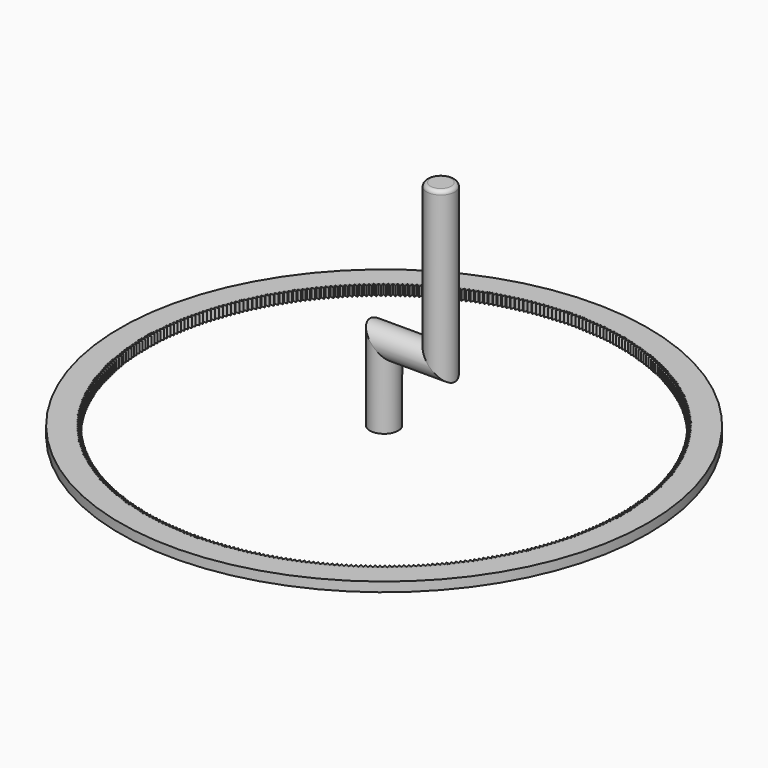
from build123d import *

# Parameters (mm, degrees)
F1_R     = 7.5
F3_R     = 2
F4_R     = 139.7
F6_DEPTH = 5
F7_COUNT = 399


# Not quite as in the source:
# - a feature names something its author has since deleted; it is built from what else it names


with BuildPart() as f2:
    # F2: sweep along a path in F0
    with BuildLine(Plane.XZ) as f2_path:
        Line((0, 0), (0, 40))
        Line((0, 40), (30, 40))
        Line((30, 40), (30, 123))
    # F1 (on Top) → F2 (sweep)
    with BuildSketch(Plane.XY):
        Circle(F1_R)
    sweep(path=f2_path.line, transition=Transition.RIGHT)

    # F3
    f3_edges = [f2.edges().sort_by_distance(p)[0] for p in [
        (22.5, 0, 123),
    ]]
    fillet(f3_edges, radius=F3_R)


with BuildPart() as f6:
    # F4 (on Top) → F6 (new body)
    with BuildSketch(Plane.XY):
        Circle(F4_R)
        with BuildLine():
            Line((127, 4.9999837018), (127, 0))
            Line((127, 0), (127, -4.9999837018))
            Line((127, -4.9999837018), (126.9015372759, -4.9999837018))
            ThreePointArc((126.9015372759, -4.9999837018), (89.8025612107, -89.8025612107), (4.9999837018, -126.9015372759))
            Line((4.9999837018, -126.9015372759), (4.9999837018, -127))
            Line((4.9999837018, -127), (0, -127))
            Line((0, -127), (-4.9999837018, -127))
            Line((-4.9999837018, -127), (-4.9999837018, -126.9015372759))
            ThreePointArc((-4.9999837018, -126.9015372759), (-89.8025612107, -89.8025612107), (-126.9015372759, -4.9999837018))
            Line((-126.9015372759, -4.9999837018), (-127, -4.9999837018))
            Line((-127, -4.9999837018), (-127, 0))
            Line((-127, 0), (-127, 4.9999837018))
            Line((-127, 4.9999837018), (-126.9015372759, 4.9999837018))
            ThreePointArc((-126.9015372759, 4.9999837018), (-89.8025612107, 89.8025612107), (-4.9999837018, 126.9015372759))
            Line((-4.9999837018, 126.9015372759), (-4.9999837018, 127))
            Line((-4.9999837018, 127), (0, 127))
            Line((0, 127), (4.9999837018, 127))
            Line((4.9999837018, 127), (4.9999837018, 126.9015372759))
            ThreePointArc((4.9999837018, 126.9015372759), (89.8025612107, 89.8025612107), (126.9015372759, 4.9999837018))
            Line((126.9015372759, 4.9999837018), (127, 4.9999837018))
        make_face(mode=Mode.SUBTRACT)
        with BuildLine():
            Line((4.9999837018, -127), (4.9999837018, -126.9015372759))
            ThreePointArc((4.9999837018, -126.9015372759), (2.5004765509, -126.9753819329), (0, -127))
            Line((0, -127), (4.9999837018, -127))
        make_face()
        with BuildLine():
            Line((-4.9999837018, -127), (0, -127))
            ThreePointArc((0, -127), (-2.5004765509, -126.9753819329), (-4.9999837018, -126.9015372759))
            Line((-4.9999837018, -126.9015372759), (-4.9999837018, -127))
        make_face()
    extrude(amount=-F6_DEPTH)


with BuildPart() as f6b:
    # F4 (on Top) → F6, piece 2 (new body)
    with BuildSketch(Plane.XY):
        Polygon((-4.75e-08, -125.2242034363), (-1.0000000475, -126.9562542439), (0.9999999525, -126.9562542439), align=None)
    extrude(amount=-F6_DEPTH)


with BuildPart() as f7_1:
    # F7: instance of F6b
    add(f6b.part.rotate(Axis((0, 0, 36.9798913598), (0, 0, 1)), 1 * 360 / F7_COUNT))


with BuildPart() as f7_2:
    # F7: instance of F6b
    add(f6b.part.rotate(Axis((0, 0, 36.9798913598), (0, 0, 1)), 2 * 360 / F7_COUNT))


with BuildPart() as f7_3:
    # F7: instance of F6b
    add(f6b.part.rotate(Axis((0, 0, 36.9798913598), (0, 0, 1)), 3 * 360 / F7_COUNT))


with BuildPart() as f7_4:
    # F7: instance of F6b
    add(f6b.part.rotate(Axis((0, 0, 36.9798913598), (0, 0, 1)), 4 * 360 / F7_COUNT))


with BuildPart() as f7_5:
    # F7: instance of F6b
    add(f6b.part.rotate(Axis((0, 0, 36.9798913598), (0, 0, 1)), 5 * 360 / F7_COUNT))


with BuildPart() as f7_6:
    # F7: instance of F6b
    add(f6b.part.rotate(Axis((0, 0, 36.9798913598), (0, 0, 1)), 6 * 360 / F7_COUNT))


with BuildPart() as f7_7:
    # F7: instance of F6b
    add(f6b.part.rotate(Axis((0, 0, 36.9798913598), (0, 0, 1)), 7 * 360 / F7_COUNT))


with BuildPart() as f7_8:
    # F7: instance of F6b
    add(f6b.part.rotate(Axis((0, 0, 36.9798913598), (0, 0, 1)), 8 * 360 / F7_COUNT))


with BuildPart() as f7_9:
    # F7: instance of F6b
    add(f6b.part.rotate(Axis((0, 0, 36.9798913598), (0, 0, 1)), 9 * 360 / F7_COUNT))


with BuildPart() as f7_10:
    # F7: instance of F6b
    add(f6b.part.rotate(Axis((0, 0, 36.9798913598), (0, 0, 1)), 10 * 360 / F7_COUNT))


with BuildPart() as f7_11:
    # F7: instance of F6b
    add(f6b.part.rotate(Axis((0, 0, 36.9798913598), (0, 0, 1)), 11 * 360 / F7_COUNT))


with BuildPart() as f7_12:
    # F7: instance of F6b
    add(f6b.part.rotate(Axis((0, 0, 36.9798913598), (0, 0, 1)), 12 * 360 / F7_COUNT))


with BuildPart() as f7_13:
    # F7: instance of F6b
    add(f6b.part.rotate(Axis((0, 0, 36.9798913598), (0, 0, 1)), 13 * 360 / F7_COUNT))


with BuildPart() as f7_14:
    # F7: instance of F6b
    add(f6b.part.rotate(Axis((0, 0, 36.9798913598), (0, 0, 1)), 14 * 360 / F7_COUNT))


with BuildPart() as f7_15:
    # F7: instance of F6b
    add(f6b.part.rotate(Axis((0, 0, 36.9798913598), (0, 0, 1)), 15 * 360 / F7_COUNT))


with BuildPart() as f7_16:
    # F7: instance of F6b
    add(f6b.part.rotate(Axis((0, 0, 36.9798913598), (0, 0, 1)), 16 * 360 / F7_COUNT))


with BuildPart() as f7_17:
    # F7: instance of F6b
    add(f6b.part.rotate(Axis((0, 0, 36.9798913598), (0, 0, 1)), 17 * 360 / F7_COUNT))


with BuildPart() as f7_18:
    # F7: instance of F6b
    add(f6b.part.rotate(Axis((0, 0, 36.9798913598), (0, 0, 1)), 18 * 360 / F7_COUNT))


with BuildPart() as f7_19:
    # F7: instance of F6b
    add(f6b.part.rotate(Axis((0, 0, 36.9798913598), (0, 0, 1)), 19 * 360 / F7_COUNT))


with BuildPart() as f7_20:
    # F7: instance of F6b
    add(f6b.part.rotate(Axis((0, 0, 36.9798913598), (0, 0, 1)), 20 * 360 / F7_COUNT))


with BuildPart() as f7_21:
    # F7: instance of F6b
    add(f6b.part.rotate(Axis((0, 0, 36.9798913598), (0, 0, 1)), 21 * 360 / F7_COUNT))


with BuildPart() as f7_22:
    # F7: instance of F6b
    add(f6b.part.rotate(Axis((0, 0, 36.9798913598), (0, 0, 1)), 22 * 360 / F7_COUNT))


with BuildPart() as f7_23:
    # F7: instance of F6b
    add(f6b.part.rotate(Axis((0, 0, 36.9798913598), (0, 0, 1)), 23 * 360 / F7_COUNT))


with BuildPart() as f7_24:
    # F7: instance of F6b
    add(f6b.part.rotate(Axis((0, 0, 36.9798913598), (0, 0, 1)), 24 * 360 / F7_COUNT))


with BuildPart() as f7_25:
    # F7: instance of F6b
    add(f6b.part.rotate(Axis((0, 0, 36.9798913598), (0, 0, 1)), 25 * 360 / F7_COUNT))


with BuildPart() as f7_26:
    # F7: instance of F6b
    add(f6b.part.rotate(Axis((0, 0, 36.9798913598), (0, 0, 1)), 26 * 360 / F7_COUNT))


with BuildPart() as f7_27:
    # F7: instance of F6b
    add(f6b.part.rotate(Axis((0, 0, 36.9798913598), (0, 0, 1)), 27 * 360 / F7_COUNT))


with BuildPart() as f7_28:
    # F7: instance of F6b
    add(f6b.part.rotate(Axis((0, 0, 36.9798913598), (0, 0, 1)), 28 * 360 / F7_COUNT))


with BuildPart() as f7_29:
    # F7: instance of F6b
    add(f6b.part.rotate(Axis((0, 0, 36.9798913598), (0, 0, 1)), 29 * 360 / F7_COUNT))


with BuildPart() as f7_30:
    # F7: instance of F6b
    add(f6b.part.rotate(Axis((0, 0, 36.9798913598), (0, 0, 1)), 30 * 360 / F7_COUNT))


with BuildPart() as f7_31:
    # F7: instance of F6b
    add(f6b.part.rotate(Axis((0, 0, 36.9798913598), (0, 0, 1)), 31 * 360 / F7_COUNT))


with BuildPart() as f7_32:
    # F7: instance of F6b
    add(f6b.part.rotate(Axis((0, 0, 36.9798913598), (0, 0, 1)), 32 * 360 / F7_COUNT))


with BuildPart() as f7_33:
    # F7: instance of F6b
    add(f6b.part.rotate(Axis((0, 0, 36.9798913598), (0, 0, 1)), 33 * 360 / F7_COUNT))


with BuildPart() as f7_34:
    # F7: instance of F6b
    add(f6b.part.rotate(Axis((0, 0, 36.9798913598), (0, 0, 1)), 34 * 360 / F7_COUNT))


with BuildPart() as f7_35:
    # F7: instance of F6b
    add(f6b.part.rotate(Axis((0, 0, 36.9798913598), (0, 0, 1)), 35 * 360 / F7_COUNT))


with BuildPart() as f7_36:
    # F7: instance of F6b
    add(f6b.part.rotate(Axis((0, 0, 36.9798913598), (0, 0, 1)), 36 * 360 / F7_COUNT))


with BuildPart() as f7_37:
    # F7: instance of F6b
    add(f6b.part.rotate(Axis((0, 0, 36.9798913598), (0, 0, 1)), 37 * 360 / F7_COUNT))


with BuildPart() as f7_38:
    # F7: instance of F6b
    add(f6b.part.rotate(Axis((0, 0, 36.9798913598), (0, 0, 1)), 38 * 360 / F7_COUNT))


with BuildPart() as f7_39:
    # F7: instance of F6b
    add(f6b.part.rotate(Axis((0, 0, 36.9798913598), (0, 0, 1)), 39 * 360 / F7_COUNT))


with BuildPart() as f7_40:
    # F7: instance of F6b
    add(f6b.part.rotate(Axis((0, 0, 36.9798913598), (0, 0, 1)), 40 * 360 / F7_COUNT))


with BuildPart() as f7_41:
    # F7: instance of F6b
    add(f6b.part.rotate(Axis((0, 0, 36.9798913598), (0, 0, 1)), 41 * 360 / F7_COUNT))


with BuildPart() as f7_42:
    # F7: instance of F6b
    add(f6b.part.rotate(Axis((0, 0, 36.9798913598), (0, 0, 1)), 42 * 360 / F7_COUNT))


with BuildPart() as f7_43:
    # F7: instance of F6b
    add(f6b.part.rotate(Axis((0, 0, 36.9798913598), (0, 0, 1)), 43 * 360 / F7_COUNT))


with BuildPart() as f7_44:
    # F7: instance of F6b
    add(f6b.part.rotate(Axis((0, 0, 36.9798913598), (0, 0, 1)), 44 * 360 / F7_COUNT))


with BuildPart() as f7_45:
    # F7: instance of F6b
    add(f6b.part.rotate(Axis((0, 0, 36.9798913598), (0, 0, 1)), 45 * 360 / F7_COUNT))


with BuildPart() as f7_46:
    # F7: instance of F6b
    add(f6b.part.rotate(Axis((0, 0, 36.9798913598), (0, 0, 1)), 46 * 360 / F7_COUNT))


with BuildPart() as f7_47:
    # F7: instance of F6b
    add(f6b.part.rotate(Axis((0, 0, 36.9798913598), (0, 0, 1)), 47 * 360 / F7_COUNT))


with BuildPart() as f7_48:
    # F7: instance of F6b
    add(f6b.part.rotate(Axis((0, 0, 36.9798913598), (0, 0, 1)), 48 * 360 / F7_COUNT))


with BuildPart() as f7_49:
    # F7: instance of F6b
    add(f6b.part.rotate(Axis((0, 0, 36.9798913598), (0, 0, 1)), 49 * 360 / F7_COUNT))


with BuildPart() as f7_50:
    # F7: instance of F6b
    add(f6b.part.rotate(Axis((0, 0, 36.9798913598), (0, 0, 1)), 50 * 360 / F7_COUNT))


with BuildPart() as f7_51:
    # F7: instance of F6b
    add(f6b.part.rotate(Axis((0, 0, 36.9798913598), (0, 0, 1)), 51 * 360 / F7_COUNT))


with BuildPart() as f7_52:
    # F7: instance of F6b
    add(f6b.part.rotate(Axis((0, 0, 36.9798913598), (0, 0, 1)), 52 * 360 / F7_COUNT))


with BuildPart() as f7_53:
    # F7: instance of F6b
    add(f6b.part.rotate(Axis((0, 0, 36.9798913598), (0, 0, 1)), 53 * 360 / F7_COUNT))


with BuildPart() as f7_54:
    # F7: instance of F6b
    add(f6b.part.rotate(Axis((0, 0, 36.9798913598), (0, 0, 1)), 54 * 360 / F7_COUNT))


with BuildPart() as f7_55:
    # F7: instance of F6b
    add(f6b.part.rotate(Axis((0, 0, 36.9798913598), (0, 0, 1)), 55 * 360 / F7_COUNT))


with BuildPart() as f7_56:
    # F7: instance of F6b
    add(f6b.part.rotate(Axis((0, 0, 36.9798913598), (0, 0, 1)), 56 * 360 / F7_COUNT))


with BuildPart() as f7_57:
    # F7: instance of F6b
    add(f6b.part.rotate(Axis((0, 0, 36.9798913598), (0, 0, 1)), 57 * 360 / F7_COUNT))


with BuildPart() as f7_58:
    # F7: instance of F6b
    add(f6b.part.rotate(Axis((0, 0, 36.9798913598), (0, 0, 1)), 58 * 360 / F7_COUNT))


with BuildPart() as f7_59:
    # F7: instance of F6b
    add(f6b.part.rotate(Axis((0, 0, 36.9798913598), (0, 0, 1)), 59 * 360 / F7_COUNT))


with BuildPart() as f7_60:
    # F7: instance of F6b
    add(f6b.part.rotate(Axis((0, 0, 36.9798913598), (0, 0, 1)), 60 * 360 / F7_COUNT))


with BuildPart() as f7_61:
    # F7: instance of F6b
    add(f6b.part.rotate(Axis((0, 0, 36.9798913598), (0, 0, 1)), 61 * 360 / F7_COUNT))


with BuildPart() as f7_62:
    # F7: instance of F6b
    add(f6b.part.rotate(Axis((0, 0, 36.9798913598), (0, 0, 1)), 62 * 360 / F7_COUNT))


with BuildPart() as f7_63:
    # F7: instance of F6b
    add(f6b.part.rotate(Axis((0, 0, 36.9798913598), (0, 0, 1)), 63 * 360 / F7_COUNT))


with BuildPart() as f7_64:
    # F7: instance of F6b
    add(f6b.part.rotate(Axis((0, 0, 36.9798913598), (0, 0, 1)), 64 * 360 / F7_COUNT))


with BuildPart() as f7_65:
    # F7: instance of F6b
    add(f6b.part.rotate(Axis((0, 0, 36.9798913598), (0, 0, 1)), 65 * 360 / F7_COUNT))


with BuildPart() as f7_66:
    # F7: instance of F6b
    add(f6b.part.rotate(Axis((0, 0, 36.9798913598), (0, 0, 1)), 66 * 360 / F7_COUNT))


with BuildPart() as f7_67:
    # F7: instance of F6b
    add(f6b.part.rotate(Axis((0, 0, 36.9798913598), (0, 0, 1)), 67 * 360 / F7_COUNT))


with BuildPart() as f7_68:
    # F7: instance of F6b
    add(f6b.part.rotate(Axis((0, 0, 36.9798913598), (0, 0, 1)), 68 * 360 / F7_COUNT))


with BuildPart() as f7_69:
    # F7: instance of F6b
    add(f6b.part.rotate(Axis((0, 0, 36.9798913598), (0, 0, 1)), 69 * 360 / F7_COUNT))


with BuildPart() as f7_70:
    # F7: instance of F6b
    add(f6b.part.rotate(Axis((0, 0, 36.9798913598), (0, 0, 1)), 70 * 360 / F7_COUNT))


with BuildPart() as f7_71:
    # F7: instance of F6b
    add(f6b.part.rotate(Axis((0, 0, 36.9798913598), (0, 0, 1)), 71 * 360 / F7_COUNT))


with BuildPart() as f7_72:
    # F7: instance of F6b
    add(f6b.part.rotate(Axis((0, 0, 36.9798913598), (0, 0, 1)), 72 * 360 / F7_COUNT))


with BuildPart() as f7_73:
    # F7: instance of F6b
    add(f6b.part.rotate(Axis((0, 0, 36.9798913598), (0, 0, 1)), 73 * 360 / F7_COUNT))


with BuildPart() as f7_74:
    # F7: instance of F6b
    add(f6b.part.rotate(Axis((0, 0, 36.9798913598), (0, 0, 1)), 74 * 360 / F7_COUNT))


with BuildPart() as f7_75:
    # F7: instance of F6b
    add(f6b.part.rotate(Axis((0, 0, 36.9798913598), (0, 0, 1)), 75 * 360 / F7_COUNT))


with BuildPart() as f7_76:
    # F7: instance of F6b
    add(f6b.part.rotate(Axis((0, 0, 36.9798913598), (0, 0, 1)), 76 * 360 / F7_COUNT))


with BuildPart() as f7_77:
    # F7: instance of F6b
    add(f6b.part.rotate(Axis((0, 0, 36.9798913598), (0, 0, 1)), 77 * 360 / F7_COUNT))


with BuildPart() as f7_78:
    # F7: instance of F6b
    add(f6b.part.rotate(Axis((0, 0, 36.9798913598), (0, 0, 1)), 78 * 360 / F7_COUNT))


with BuildPart() as f7_79:
    # F7: instance of F6b
    add(f6b.part.rotate(Axis((0, 0, 36.9798913598), (0, 0, 1)), 79 * 360 / F7_COUNT))


with BuildPart() as f7_80:
    # F7: instance of F6b
    add(f6b.part.rotate(Axis((0, 0, 36.9798913598), (0, 0, 1)), 80 * 360 / F7_COUNT))


with BuildPart() as f7_81:
    # F7: instance of F6b
    add(f6b.part.rotate(Axis((0, 0, 36.9798913598), (0, 0, 1)), 81 * 360 / F7_COUNT))


with BuildPart() as f7_82:
    # F7: instance of F6b
    add(f6b.part.rotate(Axis((0, 0, 36.9798913598), (0, 0, 1)), 82 * 360 / F7_COUNT))


with BuildPart() as f7_83:
    # F7: instance of F6b
    add(f6b.part.rotate(Axis((0, 0, 36.9798913598), (0, 0, 1)), 83 * 360 / F7_COUNT))


with BuildPart() as f7_84:
    # F7: instance of F6b
    add(f6b.part.rotate(Axis((0, 0, 36.9798913598), (0, 0, 1)), 84 * 360 / F7_COUNT))


with BuildPart() as f7_85:
    # F7: instance of F6b
    add(f6b.part.rotate(Axis((0, 0, 36.9798913598), (0, 0, 1)), 85 * 360 / F7_COUNT))


with BuildPart() as f7_86:
    # F7: instance of F6b
    add(f6b.part.rotate(Axis((0, 0, 36.9798913598), (0, 0, 1)), 86 * 360 / F7_COUNT))


with BuildPart() as f7_87:
    # F7: instance of F6b
    add(f6b.part.rotate(Axis((0, 0, 36.9798913598), (0, 0, 1)), 87 * 360 / F7_COUNT))


with BuildPart() as f7_88:
    # F7: instance of F6b
    add(f6b.part.rotate(Axis((0, 0, 36.9798913598), (0, 0, 1)), 88 * 360 / F7_COUNT))


with BuildPart() as f7_89:
    # F7: instance of F6b
    add(f6b.part.rotate(Axis((0, 0, 36.9798913598), (0, 0, 1)), 89 * 360 / F7_COUNT))


with BuildPart() as f7_90:
    # F7: instance of F6b
    add(f6b.part.rotate(Axis((0, 0, 36.9798913598), (0, 0, 1)), 90 * 360 / F7_COUNT))


with BuildPart() as f7_91:
    # F7: instance of F6b
    add(f6b.part.rotate(Axis((0, 0, 36.9798913598), (0, 0, 1)), 91 * 360 / F7_COUNT))


with BuildPart() as f7_92:
    # F7: instance of F6b
    add(f6b.part.rotate(Axis((0, 0, 36.9798913598), (0, 0, 1)), 92 * 360 / F7_COUNT))


with BuildPart() as f7_93:
    # F7: instance of F6b
    add(f6b.part.rotate(Axis((0, 0, 36.9798913598), (0, 0, 1)), 93 * 360 / F7_COUNT))


with BuildPart() as f7_94:
    # F7: instance of F6b
    add(f6b.part.rotate(Axis((0, 0, 36.9798913598), (0, 0, 1)), 94 * 360 / F7_COUNT))


with BuildPart() as f7_95:
    # F7: instance of F6b
    add(f6b.part.rotate(Axis((0, 0, 36.9798913598), (0, 0, 1)), 95 * 360 / F7_COUNT))


with BuildPart() as f7_96:
    # F7: instance of F6b
    add(f6b.part.rotate(Axis((0, 0, 36.9798913598), (0, 0, 1)), 96 * 360 / F7_COUNT))


with BuildPart() as f7_97:
    # F7: instance of F6b
    add(f6b.part.rotate(Axis((0, 0, 36.9798913598), (0, 0, 1)), 97 * 360 / F7_COUNT))


with BuildPart() as f7_98:
    # F7: instance of F6b
    add(f6b.part.rotate(Axis((0, 0, 36.9798913598), (0, 0, 1)), 98 * 360 / F7_COUNT))


with BuildPart() as f7_99:
    # F7: instance of F6b
    add(f6b.part.rotate(Axis((0, 0, 36.9798913598), (0, 0, 1)), 99 * 360 / F7_COUNT))


with BuildPart() as f7_100:
    # F7: instance of F6b
    add(f6b.part.rotate(Axis((0, 0, 36.9798913598), (0, 0, 1)), 100 * 360 / F7_COUNT))


with BuildPart() as f7_101:
    # F7: instance of F6b
    add(f6b.part.rotate(Axis((0, 0, 36.9798913598), (0, 0, 1)), 101 * 360 / F7_COUNT))


with BuildPart() as f7_102:
    # F7: instance of F6b
    add(f6b.part.rotate(Axis((0, 0, 36.9798913598), (0, 0, 1)), 102 * 360 / F7_COUNT))


with BuildPart() as f7_103:
    # F7: instance of F6b
    add(f6b.part.rotate(Axis((0, 0, 36.9798913598), (0, 0, 1)), 103 * 360 / F7_COUNT))


with BuildPart() as f7_104:
    # F7: instance of F6b
    add(f6b.part.rotate(Axis((0, 0, 36.9798913598), (0, 0, 1)), 104 * 360 / F7_COUNT))


with BuildPart() as f7_105:
    # F7: instance of F6b
    add(f6b.part.rotate(Axis((0, 0, 36.9798913598), (0, 0, 1)), 105 * 360 / F7_COUNT))


with BuildPart() as f7_106:
    # F7: instance of F6b
    add(f6b.part.rotate(Axis((0, 0, 36.9798913598), (0, 0, 1)), 106 * 360 / F7_COUNT))


with BuildPart() as f7_107:
    # F7: instance of F6b
    add(f6b.part.rotate(Axis((0, 0, 36.9798913598), (0, 0, 1)), 107 * 360 / F7_COUNT))


with BuildPart() as f7_108:
    # F7: instance of F6b
    add(f6b.part.rotate(Axis((0, 0, 36.9798913598), (0, 0, 1)), 108 * 360 / F7_COUNT))


with BuildPart() as f7_109:
    # F7: instance of F6b
    add(f6b.part.rotate(Axis((0, 0, 36.9798913598), (0, 0, 1)), 109 * 360 / F7_COUNT))


with BuildPart() as f7_110:
    # F7: instance of F6b
    add(f6b.part.rotate(Axis((0, 0, 36.9798913598), (0, 0, 1)), 110 * 360 / F7_COUNT))


with BuildPart() as f7_111:
    # F7: instance of F6b
    add(f6b.part.rotate(Axis((0, 0, 36.9798913598), (0, 0, 1)), 111 * 360 / F7_COUNT))


with BuildPart() as f7_112:
    # F7: instance of F6b
    add(f6b.part.rotate(Axis((0, 0, 36.9798913598), (0, 0, 1)), 112 * 360 / F7_COUNT))


with BuildPart() as f7_113:
    # F7: instance of F6b
    add(f6b.part.rotate(Axis((0, 0, 36.9798913598), (0, 0, 1)), 113 * 360 / F7_COUNT))


with BuildPart() as f7_114:
    # F7: instance of F6b
    add(f6b.part.rotate(Axis((0, 0, 36.9798913598), (0, 0, 1)), 114 * 360 / F7_COUNT))


with BuildPart() as f7_115:
    # F7: instance of F6b
    add(f6b.part.rotate(Axis((0, 0, 36.9798913598), (0, 0, 1)), 115 * 360 / F7_COUNT))


with BuildPart() as f7_116:
    # F7: instance of F6b
    add(f6b.part.rotate(Axis((0, 0, 36.9798913598), (0, 0, 1)), 116 * 360 / F7_COUNT))


with BuildPart() as f7_117:
    # F7: instance of F6b
    add(f6b.part.rotate(Axis((0, 0, 36.9798913598), (0, 0, 1)), 117 * 360 / F7_COUNT))


with BuildPart() as f7_118:
    # F7: instance of F6b
    add(f6b.part.rotate(Axis((0, 0, 36.9798913598), (0, 0, 1)), 118 * 360 / F7_COUNT))


with BuildPart() as f7_119:
    # F7: instance of F6b
    add(f6b.part.rotate(Axis((0, 0, 36.9798913598), (0, 0, 1)), 119 * 360 / F7_COUNT))


with BuildPart() as f7_120:
    # F7: instance of F6b
    add(f6b.part.rotate(Axis((0, 0, 36.9798913598), (0, 0, 1)), 120 * 360 / F7_COUNT))


with BuildPart() as f7_121:
    # F7: instance of F6b
    add(f6b.part.rotate(Axis((0, 0, 36.9798913598), (0, 0, 1)), 121 * 360 / F7_COUNT))


with BuildPart() as f7_122:
    # F7: instance of F6b
    add(f6b.part.rotate(Axis((0, 0, 36.9798913598), (0, 0, 1)), 122 * 360 / F7_COUNT))


with BuildPart() as f7_123:
    # F7: instance of F6b
    add(f6b.part.rotate(Axis((0, 0, 36.9798913598), (0, 0, 1)), 123 * 360 / F7_COUNT))


with BuildPart() as f7_124:
    # F7: instance of F6b
    add(f6b.part.rotate(Axis((0, 0, 36.9798913598), (0, 0, 1)), 124 * 360 / F7_COUNT))


with BuildPart() as f7_125:
    # F7: instance of F6b
    add(f6b.part.rotate(Axis((0, 0, 36.9798913598), (0, 0, 1)), 125 * 360 / F7_COUNT))


with BuildPart() as f7_126:
    # F7: instance of F6b
    add(f6b.part.rotate(Axis((0, 0, 36.9798913598), (0, 0, 1)), 126 * 360 / F7_COUNT))


with BuildPart() as f7_127:
    # F7: instance of F6b
    add(f6b.part.rotate(Axis((0, 0, 36.9798913598), (0, 0, 1)), 127 * 360 / F7_COUNT))


with BuildPart() as f7_128:
    # F7: instance of F6b
    add(f6b.part.rotate(Axis((0, 0, 36.9798913598), (0, 0, 1)), 128 * 360 / F7_COUNT))


with BuildPart() as f7_129:
    # F7: instance of F6b
    add(f6b.part.rotate(Axis((0, 0, 36.9798913598), (0, 0, 1)), 129 * 360 / F7_COUNT))


with BuildPart() as f7_130:
    # F7: instance of F6b
    add(f6b.part.rotate(Axis((0, 0, 36.9798913598), (0, 0, 1)), 130 * 360 / F7_COUNT))


with BuildPart() as f7_131:
    # F7: instance of F6b
    add(f6b.part.rotate(Axis((0, 0, 36.9798913598), (0, 0, 1)), 131 * 360 / F7_COUNT))


with BuildPart() as f7_132:
    # F7: instance of F6b
    add(f6b.part.rotate(Axis((0, 0, 36.9798913598), (0, 0, 1)), 132 * 360 / F7_COUNT))


with BuildPart() as f7_133:
    # F7: instance of F6b
    add(f6b.part.rotate(Axis((0, 0, 36.9798913598), (0, 0, 1)), 133 * 360 / F7_COUNT))


with BuildPart() as f7_134:
    # F7: instance of F6b
    add(f6b.part.rotate(Axis((0, 0, 36.9798913598), (0, 0, 1)), 134 * 360 / F7_COUNT))


with BuildPart() as f7_135:
    # F7: instance of F6b
    add(f6b.part.rotate(Axis((0, 0, 36.9798913598), (0, 0, 1)), 135 * 360 / F7_COUNT))


with BuildPart() as f7_136:
    # F7: instance of F6b
    add(f6b.part.rotate(Axis((0, 0, 36.9798913598), (0, 0, 1)), 136 * 360 / F7_COUNT))


with BuildPart() as f7_137:
    # F7: instance of F6b
    add(f6b.part.rotate(Axis((0, 0, 36.9798913598), (0, 0, 1)), 137 * 360 / F7_COUNT))


with BuildPart() as f7_138:
    # F7: instance of F6b
    add(f6b.part.rotate(Axis((0, 0, 36.9798913598), (0, 0, 1)), 138 * 360 / F7_COUNT))


with BuildPart() as f7_139:
    # F7: instance of F6b
    add(f6b.part.rotate(Axis((0, 0, 36.9798913598), (0, 0, 1)), 139 * 360 / F7_COUNT))


with BuildPart() as f7_140:
    # F7: instance of F6b
    add(f6b.part.rotate(Axis((0, 0, 36.9798913598), (0, 0, 1)), 140 * 360 / F7_COUNT))


with BuildPart() as f7_141:
    # F7: instance of F6b
    add(f6b.part.rotate(Axis((0, 0, 36.9798913598), (0, 0, 1)), 141 * 360 / F7_COUNT))


with BuildPart() as f7_142:
    # F7: instance of F6b
    add(f6b.part.rotate(Axis((0, 0, 36.9798913598), (0, 0, 1)), 142 * 360 / F7_COUNT))


with BuildPart() as f7_143:
    # F7: instance of F6b
    add(f6b.part.rotate(Axis((0, 0, 36.9798913598), (0, 0, 1)), 143 * 360 / F7_COUNT))


with BuildPart() as f7_144:
    # F7: instance of F6b
    add(f6b.part.rotate(Axis((0, 0, 36.9798913598), (0, 0, 1)), 144 * 360 / F7_COUNT))


with BuildPart() as f7_145:
    # F7: instance of F6b
    add(f6b.part.rotate(Axis((0, 0, 36.9798913598), (0, 0, 1)), 145 * 360 / F7_COUNT))


with BuildPart() as f7_146:
    # F7: instance of F6b
    add(f6b.part.rotate(Axis((0, 0, 36.9798913598), (0, 0, 1)), 146 * 360 / F7_COUNT))


with BuildPart() as f7_147:
    # F7: instance of F6b
    add(f6b.part.rotate(Axis((0, 0, 36.9798913598), (0, 0, 1)), 147 * 360 / F7_COUNT))


with BuildPart() as f7_148:
    # F7: instance of F6b
    add(f6b.part.rotate(Axis((0, 0, 36.9798913598), (0, 0, 1)), 148 * 360 / F7_COUNT))


with BuildPart() as f7_149:
    # F7: instance of F6b
    add(f6b.part.rotate(Axis((0, 0, 36.9798913598), (0, 0, 1)), 149 * 360 / F7_COUNT))


with BuildPart() as f7_150:
    # F7: instance of F6b
    add(f6b.part.rotate(Axis((0, 0, 36.9798913598), (0, 0, 1)), 150 * 360 / F7_COUNT))


with BuildPart() as f7_151:
    # F7: instance of F6b
    add(f6b.part.rotate(Axis((0, 0, 36.9798913598), (0, 0, 1)), 151 * 360 / F7_COUNT))


with BuildPart() as f7_152:
    # F7: instance of F6b
    add(f6b.part.rotate(Axis((0, 0, 36.9798913598), (0, 0, 1)), 152 * 360 / F7_COUNT))


with BuildPart() as f7_153:
    # F7: instance of F6b
    add(f6b.part.rotate(Axis((0, 0, 36.9798913598), (0, 0, 1)), 153 * 360 / F7_COUNT))


with BuildPart() as f7_154:
    # F7: instance of F6b
    add(f6b.part.rotate(Axis((0, 0, 36.9798913598), (0, 0, 1)), 154 * 360 / F7_COUNT))


with BuildPart() as f7_155:
    # F7: instance of F6b
    add(f6b.part.rotate(Axis((0, 0, 36.9798913598), (0, 0, 1)), 155 * 360 / F7_COUNT))


with BuildPart() as f7_156:
    # F7: instance of F6b
    add(f6b.part.rotate(Axis((0, 0, 36.9798913598), (0, 0, 1)), 156 * 360 / F7_COUNT))


with BuildPart() as f7_157:
    # F7: instance of F6b
    add(f6b.part.rotate(Axis((0, 0, 36.9798913598), (0, 0, 1)), 157 * 360 / F7_COUNT))


with BuildPart() as f7_158:
    # F7: instance of F6b
    add(f6b.part.rotate(Axis((0, 0, 36.9798913598), (0, 0, 1)), 158 * 360 / F7_COUNT))


with BuildPart() as f7_159:
    # F7: instance of F6b
    add(f6b.part.rotate(Axis((0, 0, 36.9798913598), (0, 0, 1)), 159 * 360 / F7_COUNT))


with BuildPart() as f7_160:
    # F7: instance of F6b
    add(f6b.part.rotate(Axis((0, 0, 36.9798913598), (0, 0, 1)), 160 * 360 / F7_COUNT))


with BuildPart() as f7_161:
    # F7: instance of F6b
    add(f6b.part.rotate(Axis((0, 0, 36.9798913598), (0, 0, 1)), 161 * 360 / F7_COUNT))


with BuildPart() as f7_162:
    # F7: instance of F6b
    add(f6b.part.rotate(Axis((0, 0, 36.9798913598), (0, 0, 1)), 162 * 360 / F7_COUNT))


with BuildPart() as f7_163:
    # F7: instance of F6b
    add(f6b.part.rotate(Axis((0, 0, 36.9798913598), (0, 0, 1)), 163 * 360 / F7_COUNT))


with BuildPart() as f7_164:
    # F7: instance of F6b
    add(f6b.part.rotate(Axis((0, 0, 36.9798913598), (0, 0, 1)), 164 * 360 / F7_COUNT))


with BuildPart() as f7_165:
    # F7: instance of F6b
    add(f6b.part.rotate(Axis((0, 0, 36.9798913598), (0, 0, 1)), 165 * 360 / F7_COUNT))


with BuildPart() as f7_166:
    # F7: instance of F6b
    add(f6b.part.rotate(Axis((0, 0, 36.9798913598), (0, 0, 1)), 166 * 360 / F7_COUNT))


with BuildPart() as f7_167:
    # F7: instance of F6b
    add(f6b.part.rotate(Axis((0, 0, 36.9798913598), (0, 0, 1)), 167 * 360 / F7_COUNT))


with BuildPart() as f7_168:
    # F7: instance of F6b
    add(f6b.part.rotate(Axis((0, 0, 36.9798913598), (0, 0, 1)), 168 * 360 / F7_COUNT))


with BuildPart() as f7_169:
    # F7: instance of F6b
    add(f6b.part.rotate(Axis((0, 0, 36.9798913598), (0, 0, 1)), 169 * 360 / F7_COUNT))


with BuildPart() as f7_170:
    # F7: instance of F6b
    add(f6b.part.rotate(Axis((0, 0, 36.9798913598), (0, 0, 1)), 170 * 360 / F7_COUNT))


with BuildPart() as f7_171:
    # F7: instance of F6b
    add(f6b.part.rotate(Axis((0, 0, 36.9798913598), (0, 0, 1)), 171 * 360 / F7_COUNT))


with BuildPart() as f7_172:
    # F7: instance of F6b
    add(f6b.part.rotate(Axis((0, 0, 36.9798913598), (0, 0, 1)), 172 * 360 / F7_COUNT))


with BuildPart() as f7_173:
    # F7: instance of F6b
    add(f6b.part.rotate(Axis((0, 0, 36.9798913598), (0, 0, 1)), 173 * 360 / F7_COUNT))


with BuildPart() as f7_174:
    # F7: instance of F6b
    add(f6b.part.rotate(Axis((0, 0, 36.9798913598), (0, 0, 1)), 174 * 360 / F7_COUNT))


with BuildPart() as f7_175:
    # F7: instance of F6b
    add(f6b.part.rotate(Axis((0, 0, 36.9798913598), (0, 0, 1)), 175 * 360 / F7_COUNT))


with BuildPart() as f7_176:
    # F7: instance of F6b
    add(f6b.part.rotate(Axis((0, 0, 36.9798913598), (0, 0, 1)), 176 * 360 / F7_COUNT))


with BuildPart() as f7_177:
    # F7: instance of F6b
    add(f6b.part.rotate(Axis((0, 0, 36.9798913598), (0, 0, 1)), 177 * 360 / F7_COUNT))


with BuildPart() as f7_178:
    # F7: instance of F6b
    add(f6b.part.rotate(Axis((0, 0, 36.9798913598), (0, 0, 1)), 178 * 360 / F7_COUNT))


with BuildPart() as f7_179:
    # F7: instance of F6b
    add(f6b.part.rotate(Axis((0, 0, 36.9798913598), (0, 0, 1)), 179 * 360 / F7_COUNT))


with BuildPart() as f7_180:
    # F7: instance of F6b
    add(f6b.part.rotate(Axis((0, 0, 36.9798913598), (0, 0, 1)), 180 * 360 / F7_COUNT))


with BuildPart() as f7_181:
    # F7: instance of F6b
    add(f6b.part.rotate(Axis((0, 0, 36.9798913598), (0, 0, 1)), 181 * 360 / F7_COUNT))


with BuildPart() as f7_182:
    # F7: instance of F6b
    add(f6b.part.rotate(Axis((0, 0, 36.9798913598), (0, 0, 1)), 182 * 360 / F7_COUNT))


with BuildPart() as f7_183:
    # F7: instance of F6b
    add(f6b.part.rotate(Axis((0, 0, 36.9798913598), (0, 0, 1)), 183 * 360 / F7_COUNT))


with BuildPart() as f7_184:
    # F7: instance of F6b
    add(f6b.part.rotate(Axis((0, 0, 36.9798913598), (0, 0, 1)), 184 * 360 / F7_COUNT))


with BuildPart() as f7_185:
    # F7: instance of F6b
    add(f6b.part.rotate(Axis((0, 0, 36.9798913598), (0, 0, 1)), 185 * 360 / F7_COUNT))


with BuildPart() as f7_186:
    # F7: instance of F6b
    add(f6b.part.rotate(Axis((0, 0, 36.9798913598), (0, 0, 1)), 186 * 360 / F7_COUNT))


with BuildPart() as f7_187:
    # F7: instance of F6b
    add(f6b.part.rotate(Axis((0, 0, 36.9798913598), (0, 0, 1)), 187 * 360 / F7_COUNT))


with BuildPart() as f7_188:
    # F7: instance of F6b
    add(f6b.part.rotate(Axis((0, 0, 36.9798913598), (0, 0, 1)), 188 * 360 / F7_COUNT))


with BuildPart() as f7_189:
    # F7: instance of F6b
    add(f6b.part.rotate(Axis((0, 0, 36.9798913598), (0, 0, 1)), 189 * 360 / F7_COUNT))


with BuildPart() as f7_190:
    # F7: instance of F6b
    add(f6b.part.rotate(Axis((0, 0, 36.9798913598), (0, 0, 1)), 190 * 360 / F7_COUNT))


with BuildPart() as f7_191:
    # F7: instance of F6b
    add(f6b.part.rotate(Axis((0, 0, 36.9798913598), (0, 0, 1)), 191 * 360 / F7_COUNT))


with BuildPart() as f7_192:
    # F7: instance of F6b
    add(f6b.part.rotate(Axis((0, 0, 36.9798913598), (0, 0, 1)), 192 * 360 / F7_COUNT))


with BuildPart() as f7_193:
    # F7: instance of F6b
    add(f6b.part.rotate(Axis((0, 0, 36.9798913598), (0, 0, 1)), 193 * 360 / F7_COUNT))


with BuildPart() as f7_194:
    # F7: instance of F6b
    add(f6b.part.rotate(Axis((0, 0, 36.9798913598), (0, 0, 1)), 194 * 360 / F7_COUNT))


with BuildPart() as f7_195:
    # F7: instance of F6b
    add(f6b.part.rotate(Axis((0, 0, 36.9798913598), (0, 0, 1)), 195 * 360 / F7_COUNT))


with BuildPart() as f7_196:
    # F7: instance of F6b
    add(f6b.part.rotate(Axis((0, 0, 36.9798913598), (0, 0, 1)), 196 * 360 / F7_COUNT))


with BuildPart() as f7_197:
    # F7: instance of F6b
    add(f6b.part.rotate(Axis((0, 0, 36.9798913598), (0, 0, 1)), 197 * 360 / F7_COUNT))


with BuildPart() as f7_198:
    # F7: instance of F6b
    add(f6b.part.rotate(Axis((0, 0, 36.9798913598), (0, 0, 1)), 198 * 360 / F7_COUNT))


with BuildPart() as f7_199:
    # F7: instance of F6b
    add(f6b.part.rotate(Axis((0, 0, 36.9798913598), (0, 0, 1)), 199 * 360 / F7_COUNT))


with BuildPart() as f7_200:
    # F7: instance of F6b
    add(f6b.part.rotate(Axis((0, 0, 36.9798913598), (0, 0, 1)), 200 * 360 / F7_COUNT))


with BuildPart() as f7_201:
    # F7: instance of F6b
    add(f6b.part.rotate(Axis((0, 0, 36.9798913598), (0, 0, 1)), 201 * 360 / F7_COUNT))


with BuildPart() as f7_202:
    # F7: instance of F6b
    add(f6b.part.rotate(Axis((0, 0, 36.9798913598), (0, 0, 1)), 202 * 360 / F7_COUNT))


with BuildPart() as f7_203:
    # F7: instance of F6b
    add(f6b.part.rotate(Axis((0, 0, 36.9798913598), (0, 0, 1)), 203 * 360 / F7_COUNT))


with BuildPart() as f7_204:
    # F7: instance of F6b
    add(f6b.part.rotate(Axis((0, 0, 36.9798913598), (0, 0, 1)), 204 * 360 / F7_COUNT))


with BuildPart() as f7_205:
    # F7: instance of F6b
    add(f6b.part.rotate(Axis((0, 0, 36.9798913598), (0, 0, 1)), 205 * 360 / F7_COUNT))


with BuildPart() as f7_206:
    # F7: instance of F6b
    add(f6b.part.rotate(Axis((0, 0, 36.9798913598), (0, 0, 1)), 206 * 360 / F7_COUNT))


with BuildPart() as f7_207:
    # F7: instance of F6b
    add(f6b.part.rotate(Axis((0, 0, 36.9798913598), (0, 0, 1)), 207 * 360 / F7_COUNT))


with BuildPart() as f7_208:
    # F7: instance of F6b
    add(f6b.part.rotate(Axis((0, 0, 36.9798913598), (0, 0, 1)), 208 * 360 / F7_COUNT))


with BuildPart() as f7_209:
    # F7: instance of F6b
    add(f6b.part.rotate(Axis((0, 0, 36.9798913598), (0, 0, 1)), 209 * 360 / F7_COUNT))


with BuildPart() as f7_210:
    # F7: instance of F6b
    add(f6b.part.rotate(Axis((0, 0, 36.9798913598), (0, 0, 1)), 210 * 360 / F7_COUNT))


with BuildPart() as f7_211:
    # F7: instance of F6b
    add(f6b.part.rotate(Axis((0, 0, 36.9798913598), (0, 0, 1)), 211 * 360 / F7_COUNT))


with BuildPart() as f7_212:
    # F7: instance of F6b
    add(f6b.part.rotate(Axis((0, 0, 36.9798913598), (0, 0, 1)), 212 * 360 / F7_COUNT))


with BuildPart() as f7_213:
    # F7: instance of F6b
    add(f6b.part.rotate(Axis((0, 0, 36.9798913598), (0, 0, 1)), 213 * 360 / F7_COUNT))


with BuildPart() as f7_214:
    # F7: instance of F6b
    add(f6b.part.rotate(Axis((0, 0, 36.9798913598), (0, 0, 1)), 214 * 360 / F7_COUNT))


with BuildPart() as f7_215:
    # F7: instance of F6b
    add(f6b.part.rotate(Axis((0, 0, 36.9798913598), (0, 0, 1)), 215 * 360 / F7_COUNT))


with BuildPart() as f7_216:
    # F7: instance of F6b
    add(f6b.part.rotate(Axis((0, 0, 36.9798913598), (0, 0, 1)), 216 * 360 / F7_COUNT))


with BuildPart() as f7_217:
    # F7: instance of F6b
    add(f6b.part.rotate(Axis((0, 0, 36.9798913598), (0, 0, 1)), 217 * 360 / F7_COUNT))


with BuildPart() as f7_218:
    # F7: instance of F6b
    add(f6b.part.rotate(Axis((0, 0, 36.9798913598), (0, 0, 1)), 218 * 360 / F7_COUNT))


with BuildPart() as f7_219:
    # F7: instance of F6b
    add(f6b.part.rotate(Axis((0, 0, 36.9798913598), (0, 0, 1)), 219 * 360 / F7_COUNT))


with BuildPart() as f7_220:
    # F7: instance of F6b
    add(f6b.part.rotate(Axis((0, 0, 36.9798913598), (0, 0, 1)), 220 * 360 / F7_COUNT))


with BuildPart() as f7_221:
    # F7: instance of F6b
    add(f6b.part.rotate(Axis((0, 0, 36.9798913598), (0, 0, 1)), 221 * 360 / F7_COUNT))


with BuildPart() as f7_222:
    # F7: instance of F6b
    add(f6b.part.rotate(Axis((0, 0, 36.9798913598), (0, 0, 1)), 222 * 360 / F7_COUNT))


with BuildPart() as f7_223:
    # F7: instance of F6b
    add(f6b.part.rotate(Axis((0, 0, 36.9798913598), (0, 0, 1)), 223 * 360 / F7_COUNT))


with BuildPart() as f7_224:
    # F7: instance of F6b
    add(f6b.part.rotate(Axis((0, 0, 36.9798913598), (0, 0, 1)), 224 * 360 / F7_COUNT))


with BuildPart() as f7_225:
    # F7: instance of F6b
    add(f6b.part.rotate(Axis((0, 0, 36.9798913598), (0, 0, 1)), 225 * 360 / F7_COUNT))


with BuildPart() as f7_226:
    # F7: instance of F6b
    add(f6b.part.rotate(Axis((0, 0, 36.9798913598), (0, 0, 1)), 226 * 360 / F7_COUNT))


with BuildPart() as f7_227:
    # F7: instance of F6b
    add(f6b.part.rotate(Axis((0, 0, 36.9798913598), (0, 0, 1)), 227 * 360 / F7_COUNT))


with BuildPart() as f7_228:
    # F7: instance of F6b
    add(f6b.part.rotate(Axis((0, 0, 36.9798913598), (0, 0, 1)), 228 * 360 / F7_COUNT))


with BuildPart() as f7_229:
    # F7: instance of F6b
    add(f6b.part.rotate(Axis((0, 0, 36.9798913598), (0, 0, 1)), 229 * 360 / F7_COUNT))


with BuildPart() as f7_230:
    # F7: instance of F6b
    add(f6b.part.rotate(Axis((0, 0, 36.9798913598), (0, 0, 1)), 230 * 360 / F7_COUNT))


with BuildPart() as f7_231:
    # F7: instance of F6b
    add(f6b.part.rotate(Axis((0, 0, 36.9798913598), (0, 0, 1)), 231 * 360 / F7_COUNT))


with BuildPart() as f7_232:
    # F7: instance of F6b
    add(f6b.part.rotate(Axis((0, 0, 36.9798913598), (0, 0, 1)), 232 * 360 / F7_COUNT))


with BuildPart() as f7_233:
    # F7: instance of F6b
    add(f6b.part.rotate(Axis((0, 0, 36.9798913598), (0, 0, 1)), 233 * 360 / F7_COUNT))


with BuildPart() as f7_234:
    # F7: instance of F6b
    add(f6b.part.rotate(Axis((0, 0, 36.9798913598), (0, 0, 1)), 234 * 360 / F7_COUNT))


with BuildPart() as f7_235:
    # F7: instance of F6b
    add(f6b.part.rotate(Axis((0, 0, 36.9798913598), (0, 0, 1)), 235 * 360 / F7_COUNT))


with BuildPart() as f7_236:
    # F7: instance of F6b
    add(f6b.part.rotate(Axis((0, 0, 36.9798913598), (0, 0, 1)), 236 * 360 / F7_COUNT))


with BuildPart() as f7_237:
    # F7: instance of F6b
    add(f6b.part.rotate(Axis((0, 0, 36.9798913598), (0, 0, 1)), 237 * 360 / F7_COUNT))


with BuildPart() as f7_238:
    # F7: instance of F6b
    add(f6b.part.rotate(Axis((0, 0, 36.9798913598), (0, 0, 1)), 238 * 360 / F7_COUNT))


with BuildPart() as f7_239:
    # F7: instance of F6b
    add(f6b.part.rotate(Axis((0, 0, 36.9798913598), (0, 0, 1)), 239 * 360 / F7_COUNT))


with BuildPart() as f7_240:
    # F7: instance of F6b
    add(f6b.part.rotate(Axis((0, 0, 36.9798913598), (0, 0, 1)), 240 * 360 / F7_COUNT))


with BuildPart() as f7_241:
    # F7: instance of F6b
    add(f6b.part.rotate(Axis((0, 0, 36.9798913598), (0, 0, 1)), 241 * 360 / F7_COUNT))


with BuildPart() as f7_242:
    # F7: instance of F6b
    add(f6b.part.rotate(Axis((0, 0, 36.9798913598), (0, 0, 1)), 242 * 360 / F7_COUNT))


with BuildPart() as f7_243:
    # F7: instance of F6b
    add(f6b.part.rotate(Axis((0, 0, 36.9798913598), (0, 0, 1)), 243 * 360 / F7_COUNT))


with BuildPart() as f7_244:
    # F7: instance of F6b
    add(f6b.part.rotate(Axis((0, 0, 36.9798913598), (0, 0, 1)), 244 * 360 / F7_COUNT))


with BuildPart() as f7_245:
    # F7: instance of F6b
    add(f6b.part.rotate(Axis((0, 0, 36.9798913598), (0, 0, 1)), 245 * 360 / F7_COUNT))


with BuildPart() as f7_246:
    # F7: instance of F6b
    add(f6b.part.rotate(Axis((0, 0, 36.9798913598), (0, 0, 1)), 246 * 360 / F7_COUNT))


with BuildPart() as f7_247:
    # F7: instance of F6b
    add(f6b.part.rotate(Axis((0, 0, 36.9798913598), (0, 0, 1)), 247 * 360 / F7_COUNT))


with BuildPart() as f7_248:
    # F7: instance of F6b
    add(f6b.part.rotate(Axis((0, 0, 36.9798913598), (0, 0, 1)), 248 * 360 / F7_COUNT))


with BuildPart() as f7_249:
    # F7: instance of F6b
    add(f6b.part.rotate(Axis((0, 0, 36.9798913598), (0, 0, 1)), 249 * 360 / F7_COUNT))


with BuildPart() as f7_250:
    # F7: instance of F6b
    add(f6b.part.rotate(Axis((0, 0, 36.9798913598), (0, 0, 1)), 250 * 360 / F7_COUNT))


with BuildPart() as f7_251:
    # F7: instance of F6b
    add(f6b.part.rotate(Axis((0, 0, 36.9798913598), (0, 0, 1)), 251 * 360 / F7_COUNT))


with BuildPart() as f7_252:
    # F7: instance of F6b
    add(f6b.part.rotate(Axis((0, 0, 36.9798913598), (0, 0, 1)), 252 * 360 / F7_COUNT))


with BuildPart() as f7_253:
    # F7: instance of F6b
    add(f6b.part.rotate(Axis((0, 0, 36.9798913598), (0, 0, 1)), 253 * 360 / F7_COUNT))


with BuildPart() as f7_254:
    # F7: instance of F6b
    add(f6b.part.rotate(Axis((0, 0, 36.9798913598), (0, 0, 1)), 254 * 360 / F7_COUNT))


with BuildPart() as f7_255:
    # F7: instance of F6b
    add(f6b.part.rotate(Axis((0, 0, 36.9798913598), (0, 0, 1)), 255 * 360 / F7_COUNT))


with BuildPart() as f7_256:
    # F7: instance of F6b
    add(f6b.part.rotate(Axis((0, 0, 36.9798913598), (0, 0, 1)), 256 * 360 / F7_COUNT))


with BuildPart() as f7_257:
    # F7: instance of F6b
    add(f6b.part.rotate(Axis((0, 0, 36.9798913598), (0, 0, 1)), 257 * 360 / F7_COUNT))


with BuildPart() as f7_258:
    # F7: instance of F6b
    add(f6b.part.rotate(Axis((0, 0, 36.9798913598), (0, 0, 1)), 258 * 360 / F7_COUNT))


with BuildPart() as f7_259:
    # F7: instance of F6b
    add(f6b.part.rotate(Axis((0, 0, 36.9798913598), (0, 0, 1)), 259 * 360 / F7_COUNT))


with BuildPart() as f7_260:
    # F7: instance of F6b
    add(f6b.part.rotate(Axis((0, 0, 36.9798913598), (0, 0, 1)), 260 * 360 / F7_COUNT))


with BuildPart() as f7_261:
    # F7: instance of F6b
    add(f6b.part.rotate(Axis((0, 0, 36.9798913598), (0, 0, 1)), 261 * 360 / F7_COUNT))


with BuildPart() as f7_262:
    # F7: instance of F6b
    add(f6b.part.rotate(Axis((0, 0, 36.9798913598), (0, 0, 1)), 262 * 360 / F7_COUNT))


with BuildPart() as f7_263:
    # F7: instance of F6b
    add(f6b.part.rotate(Axis((0, 0, 36.9798913598), (0, 0, 1)), 263 * 360 / F7_COUNT))


with BuildPart() as f7_264:
    # F7: instance of F6b
    add(f6b.part.rotate(Axis((0, 0, 36.9798913598), (0, 0, 1)), 264 * 360 / F7_COUNT))


with BuildPart() as f7_265:
    # F7: instance of F6b
    add(f6b.part.rotate(Axis((0, 0, 36.9798913598), (0, 0, 1)), 265 * 360 / F7_COUNT))


with BuildPart() as f7_266:
    # F7: instance of F6b
    add(f6b.part.rotate(Axis((0, 0, 36.9798913598), (0, 0, 1)), 266 * 360 / F7_COUNT))


with BuildPart() as f7_267:
    # F7: instance of F6b
    add(f6b.part.rotate(Axis((0, 0, 36.9798913598), (0, 0, 1)), 267 * 360 / F7_COUNT))


with BuildPart() as f7_268:
    # F7: instance of F6b
    add(f6b.part.rotate(Axis((0, 0, 36.9798913598), (0, 0, 1)), 268 * 360 / F7_COUNT))


with BuildPart() as f7_269:
    # F7: instance of F6b
    add(f6b.part.rotate(Axis((0, 0, 36.9798913598), (0, 0, 1)), 269 * 360 / F7_COUNT))


with BuildPart() as f7_270:
    # F7: instance of F6b
    add(f6b.part.rotate(Axis((0, 0, 36.9798913598), (0, 0, 1)), 270 * 360 / F7_COUNT))


with BuildPart() as f7_271:
    # F7: instance of F6b
    add(f6b.part.rotate(Axis((0, 0, 36.9798913598), (0, 0, 1)), 271 * 360 / F7_COUNT))


with BuildPart() as f7_272:
    # F7: instance of F6b
    add(f6b.part.rotate(Axis((0, 0, 36.9798913598), (0, 0, 1)), 272 * 360 / F7_COUNT))


with BuildPart() as f7_273:
    # F7: instance of F6b
    add(f6b.part.rotate(Axis((0, 0, 36.9798913598), (0, 0, 1)), 273 * 360 / F7_COUNT))


with BuildPart() as f7_274:
    # F7: instance of F6b
    add(f6b.part.rotate(Axis((0, 0, 36.9798913598), (0, 0, 1)), 274 * 360 / F7_COUNT))


with BuildPart() as f7_275:
    # F7: instance of F6b
    add(f6b.part.rotate(Axis((0, 0, 36.9798913598), (0, 0, 1)), 275 * 360 / F7_COUNT))


with BuildPart() as f7_276:
    # F7: instance of F6b
    add(f6b.part.rotate(Axis((0, 0, 36.9798913598), (0, 0, 1)), 276 * 360 / F7_COUNT))


with BuildPart() as f7_277:
    # F7: instance of F6b
    add(f6b.part.rotate(Axis((0, 0, 36.9798913598), (0, 0, 1)), 277 * 360 / F7_COUNT))


with BuildPart() as f7_278:
    # F7: instance of F6b
    add(f6b.part.rotate(Axis((0, 0, 36.9798913598), (0, 0, 1)), 278 * 360 / F7_COUNT))


with BuildPart() as f7_279:
    # F7: instance of F6b
    add(f6b.part.rotate(Axis((0, 0, 36.9798913598), (0, 0, 1)), 279 * 360 / F7_COUNT))


with BuildPart() as f7_280:
    # F7: instance of F6b
    add(f6b.part.rotate(Axis((0, 0, 36.9798913598), (0, 0, 1)), 280 * 360 / F7_COUNT))


with BuildPart() as f7_281:
    # F7: instance of F6b
    add(f6b.part.rotate(Axis((0, 0, 36.9798913598), (0, 0, 1)), 281 * 360 / F7_COUNT))


with BuildPart() as f7_282:
    # F7: instance of F6b
    add(f6b.part.rotate(Axis((0, 0, 36.9798913598), (0, 0, 1)), 282 * 360 / F7_COUNT))


with BuildPart() as f7_283:
    # F7: instance of F6b
    add(f6b.part.rotate(Axis((0, 0, 36.9798913598), (0, 0, 1)), 283 * 360 / F7_COUNT))


with BuildPart() as f7_284:
    # F7: instance of F6b
    add(f6b.part.rotate(Axis((0, 0, 36.9798913598), (0, 0, 1)), 284 * 360 / F7_COUNT))


with BuildPart() as f7_285:
    # F7: instance of F6b
    add(f6b.part.rotate(Axis((0, 0, 36.9798913598), (0, 0, 1)), 285 * 360 / F7_COUNT))


with BuildPart() as f7_286:
    # F7: instance of F6b
    add(f6b.part.rotate(Axis((0, 0, 36.9798913598), (0, 0, 1)), 286 * 360 / F7_COUNT))


with BuildPart() as f7_287:
    # F7: instance of F6b
    add(f6b.part.rotate(Axis((0, 0, 36.9798913598), (0, 0, 1)), 287 * 360 / F7_COUNT))


with BuildPart() as f7_288:
    # F7: instance of F6b
    add(f6b.part.rotate(Axis((0, 0, 36.9798913598), (0, 0, 1)), 288 * 360 / F7_COUNT))


with BuildPart() as f7_289:
    # F7: instance of F6b
    add(f6b.part.rotate(Axis((0, 0, 36.9798913598), (0, 0, 1)), 289 * 360 / F7_COUNT))


with BuildPart() as f7_290:
    # F7: instance of F6b
    add(f6b.part.rotate(Axis((0, 0, 36.9798913598), (0, 0, 1)), 290 * 360 / F7_COUNT))


with BuildPart() as f7_291:
    # F7: instance of F6b
    add(f6b.part.rotate(Axis((0, 0, 36.9798913598), (0, 0, 1)), 291 * 360 / F7_COUNT))


with BuildPart() as f7_292:
    # F7: instance of F6b
    add(f6b.part.rotate(Axis((0, 0, 36.9798913598), (0, 0, 1)), 292 * 360 / F7_COUNT))


with BuildPart() as f7_293:
    # F7: instance of F6b
    add(f6b.part.rotate(Axis((0, 0, 36.9798913598), (0, 0, 1)), 293 * 360 / F7_COUNT))


with BuildPart() as f7_294:
    # F7: instance of F6b
    add(f6b.part.rotate(Axis((0, 0, 36.9798913598), (0, 0, 1)), 294 * 360 / F7_COUNT))


with BuildPart() as f7_295:
    # F7: instance of F6b
    add(f6b.part.rotate(Axis((0, 0, 36.9798913598), (0, 0, 1)), 295 * 360 / F7_COUNT))


with BuildPart() as f7_296:
    # F7: instance of F6b
    add(f6b.part.rotate(Axis((0, 0, 36.9798913598), (0, 0, 1)), 296 * 360 / F7_COUNT))


with BuildPart() as f7_297:
    # F7: instance of F6b
    add(f6b.part.rotate(Axis((0, 0, 36.9798913598), (0, 0, 1)), 297 * 360 / F7_COUNT))


with BuildPart() as f7_298:
    # F7: instance of F6b
    add(f6b.part.rotate(Axis((0, 0, 36.9798913598), (0, 0, 1)), 298 * 360 / F7_COUNT))


with BuildPart() as f7_299:
    # F7: instance of F6b
    add(f6b.part.rotate(Axis((0, 0, 36.9798913598), (0, 0, 1)), 299 * 360 / F7_COUNT))


with BuildPart() as f7_300:
    # F7: instance of F6b
    add(f6b.part.rotate(Axis((0, 0, 36.9798913598), (0, 0, 1)), 300 * 360 / F7_COUNT))


with BuildPart() as f7_301:
    # F7: instance of F6b
    add(f6b.part.rotate(Axis((0, 0, 36.9798913598), (0, 0, 1)), 301 * 360 / F7_COUNT))


with BuildPart() as f7_302:
    # F7: instance of F6b
    add(f6b.part.rotate(Axis((0, 0, 36.9798913598), (0, 0, 1)), 302 * 360 / F7_COUNT))


with BuildPart() as f7_303:
    # F7: instance of F6b
    add(f6b.part.rotate(Axis((0, 0, 36.9798913598), (0, 0, 1)), 303 * 360 / F7_COUNT))


with BuildPart() as f7_304:
    # F7: instance of F6b
    add(f6b.part.rotate(Axis((0, 0, 36.9798913598), (0, 0, 1)), 304 * 360 / F7_COUNT))


with BuildPart() as f7_305:
    # F7: instance of F6b
    add(f6b.part.rotate(Axis((0, 0, 36.9798913598), (0, 0, 1)), 305 * 360 / F7_COUNT))


with BuildPart() as f7_306:
    # F7: instance of F6b
    add(f6b.part.rotate(Axis((0, 0, 36.9798913598), (0, 0, 1)), 306 * 360 / F7_COUNT))


with BuildPart() as f7_307:
    # F7: instance of F6b
    add(f6b.part.rotate(Axis((0, 0, 36.9798913598), (0, 0, 1)), 307 * 360 / F7_COUNT))


with BuildPart() as f7_308:
    # F7: instance of F6b
    add(f6b.part.rotate(Axis((0, 0, 36.9798913598), (0, 0, 1)), 308 * 360 / F7_COUNT))


with BuildPart() as f7_309:
    # F7: instance of F6b
    add(f6b.part.rotate(Axis((0, 0, 36.9798913598), (0, 0, 1)), 309 * 360 / F7_COUNT))


with BuildPart() as f7_310:
    # F7: instance of F6b
    add(f6b.part.rotate(Axis((0, 0, 36.9798913598), (0, 0, 1)), 310 * 360 / F7_COUNT))


with BuildPart() as f7_311:
    # F7: instance of F6b
    add(f6b.part.rotate(Axis((0, 0, 36.9798913598), (0, 0, 1)), 311 * 360 / F7_COUNT))


with BuildPart() as f7_312:
    # F7: instance of F6b
    add(f6b.part.rotate(Axis((0, 0, 36.9798913598), (0, 0, 1)), 312 * 360 / F7_COUNT))


with BuildPart() as f7_313:
    # F7: instance of F6b
    add(f6b.part.rotate(Axis((0, 0, 36.9798913598), (0, 0, 1)), 313 * 360 / F7_COUNT))


with BuildPart() as f7_314:
    # F7: instance of F6b
    add(f6b.part.rotate(Axis((0, 0, 36.9798913598), (0, 0, 1)), 314 * 360 / F7_COUNT))


with BuildPart() as f7_315:
    # F7: instance of F6b
    add(f6b.part.rotate(Axis((0, 0, 36.9798913598), (0, 0, 1)), 315 * 360 / F7_COUNT))


with BuildPart() as f7_316:
    # F7: instance of F6b
    add(f6b.part.rotate(Axis((0, 0, 36.9798913598), (0, 0, 1)), 316 * 360 / F7_COUNT))


with BuildPart() as f7_317:
    # F7: instance of F6b
    add(f6b.part.rotate(Axis((0, 0, 36.9798913598), (0, 0, 1)), 317 * 360 / F7_COUNT))


with BuildPart() as f7_318:
    # F7: instance of F6b
    add(f6b.part.rotate(Axis((0, 0, 36.9798913598), (0, 0, 1)), 318 * 360 / F7_COUNT))


with BuildPart() as f7_319:
    # F7: instance of F6b
    add(f6b.part.rotate(Axis((0, 0, 36.9798913598), (0, 0, 1)), 319 * 360 / F7_COUNT))


with BuildPart() as f7_320:
    # F7: instance of F6b
    add(f6b.part.rotate(Axis((0, 0, 36.9798913598), (0, 0, 1)), 320 * 360 / F7_COUNT))


with BuildPart() as f7_321:
    # F7: instance of F6b
    add(f6b.part.rotate(Axis((0, 0, 36.9798913598), (0, 0, 1)), 321 * 360 / F7_COUNT))


with BuildPart() as f7_322:
    # F7: instance of F6b
    add(f6b.part.rotate(Axis((0, 0, 36.9798913598), (0, 0, 1)), 322 * 360 / F7_COUNT))


with BuildPart() as f7_323:
    # F7: instance of F6b
    add(f6b.part.rotate(Axis((0, 0, 36.9798913598), (0, 0, 1)), 323 * 360 / F7_COUNT))


with BuildPart() as f7_324:
    # F7: instance of F6b
    add(f6b.part.rotate(Axis((0, 0, 36.9798913598), (0, 0, 1)), 324 * 360 / F7_COUNT))


with BuildPart() as f7_325:
    # F7: instance of F6b
    add(f6b.part.rotate(Axis((0, 0, 36.9798913598), (0, 0, 1)), 325 * 360 / F7_COUNT))


with BuildPart() as f7_326:
    # F7: instance of F6b
    add(f6b.part.rotate(Axis((0, 0, 36.9798913598), (0, 0, 1)), 326 * 360 / F7_COUNT))


with BuildPart() as f7_327:
    # F7: instance of F6b
    add(f6b.part.rotate(Axis((0, 0, 36.9798913598), (0, 0, 1)), 327 * 360 / F7_COUNT))


with BuildPart() as f7_328:
    # F7: instance of F6b
    add(f6b.part.rotate(Axis((0, 0, 36.9798913598), (0, 0, 1)), 328 * 360 / F7_COUNT))


with BuildPart() as f7_329:
    # F7: instance of F6b
    add(f6b.part.rotate(Axis((0, 0, 36.9798913598), (0, 0, 1)), 329 * 360 / F7_COUNT))


with BuildPart() as f7_330:
    # F7: instance of F6b
    add(f6b.part.rotate(Axis((0, 0, 36.9798913598), (0, 0, 1)), 330 * 360 / F7_COUNT))


with BuildPart() as f7_331:
    # F7: instance of F6b
    add(f6b.part.rotate(Axis((0, 0, 36.9798913598), (0, 0, 1)), 331 * 360 / F7_COUNT))


with BuildPart() as f7_332:
    # F7: instance of F6b
    add(f6b.part.rotate(Axis((0, 0, 36.9798913598), (0, 0, 1)), 332 * 360 / F7_COUNT))


with BuildPart() as f7_333:
    # F7: instance of F6b
    add(f6b.part.rotate(Axis((0, 0, 36.9798913598), (0, 0, 1)), 333 * 360 / F7_COUNT))


with BuildPart() as f7_334:
    # F7: instance of F6b
    add(f6b.part.rotate(Axis((0, 0, 36.9798913598), (0, 0, 1)), 334 * 360 / F7_COUNT))


with BuildPart() as f7_335:
    # F7: instance of F6b
    add(f6b.part.rotate(Axis((0, 0, 36.9798913598), (0, 0, 1)), 335 * 360 / F7_COUNT))


with BuildPart() as f7_336:
    # F7: instance of F6b
    add(f6b.part.rotate(Axis((0, 0, 36.9798913598), (0, 0, 1)), 336 * 360 / F7_COUNT))


with BuildPart() as f7_337:
    # F7: instance of F6b
    add(f6b.part.rotate(Axis((0, 0, 36.9798913598), (0, 0, 1)), 337 * 360 / F7_COUNT))


with BuildPart() as f7_338:
    # F7: instance of F6b
    add(f6b.part.rotate(Axis((0, 0, 36.9798913598), (0, 0, 1)), 338 * 360 / F7_COUNT))


with BuildPart() as f7_339:
    # F7: instance of F6b
    add(f6b.part.rotate(Axis((0, 0, 36.9798913598), (0, 0, 1)), 339 * 360 / F7_COUNT))


with BuildPart() as f7_340:
    # F7: instance of F6b
    add(f6b.part.rotate(Axis((0, 0, 36.9798913598), (0, 0, 1)), 340 * 360 / F7_COUNT))


with BuildPart() as f7_341:
    # F7: instance of F6b
    add(f6b.part.rotate(Axis((0, 0, 36.9798913598), (0, 0, 1)), 341 * 360 / F7_COUNT))


with BuildPart() as f7_342:
    # F7: instance of F6b
    add(f6b.part.rotate(Axis((0, 0, 36.9798913598), (0, 0, 1)), 342 * 360 / F7_COUNT))


with BuildPart() as f7_343:
    # F7: instance of F6b
    add(f6b.part.rotate(Axis((0, 0, 36.9798913598), (0, 0, 1)), 343 * 360 / F7_COUNT))


with BuildPart() as f7_344:
    # F7: instance of F6b
    add(f6b.part.rotate(Axis((0, 0, 36.9798913598), (0, 0, 1)), 344 * 360 / F7_COUNT))


with BuildPart() as f7_345:
    # F7: instance of F6b
    add(f6b.part.rotate(Axis((0, 0, 36.9798913598), (0, 0, 1)), 345 * 360 / F7_COUNT))


with BuildPart() as f7_346:
    # F7: instance of F6b
    add(f6b.part.rotate(Axis((0, 0, 36.9798913598), (0, 0, 1)), 346 * 360 / F7_COUNT))


with BuildPart() as f7_347:
    # F7: instance of F6b
    add(f6b.part.rotate(Axis((0, 0, 36.9798913598), (0, 0, 1)), 347 * 360 / F7_COUNT))


with BuildPart() as f7_348:
    # F7: instance of F6b
    add(f6b.part.rotate(Axis((0, 0, 36.9798913598), (0, 0, 1)), 348 * 360 / F7_COUNT))


with BuildPart() as f7_349:
    # F7: instance of F6b
    add(f6b.part.rotate(Axis((0, 0, 36.9798913598), (0, 0, 1)), 349 * 360 / F7_COUNT))


with BuildPart() as f7_350:
    # F7: instance of F6b
    add(f6b.part.rotate(Axis((0, 0, 36.9798913598), (0, 0, 1)), 350 * 360 / F7_COUNT))


with BuildPart() as f7_351:
    # F7: instance of F6b
    add(f6b.part.rotate(Axis((0, 0, 36.9798913598), (0, 0, 1)), 351 * 360 / F7_COUNT))


with BuildPart() as f7_352:
    # F7: instance of F6b
    add(f6b.part.rotate(Axis((0, 0, 36.9798913598), (0, 0, 1)), 352 * 360 / F7_COUNT))


with BuildPart() as f7_353:
    # F7: instance of F6b
    add(f6b.part.rotate(Axis((0, 0, 36.9798913598), (0, 0, 1)), 353 * 360 / F7_COUNT))


with BuildPart() as f7_354:
    # F7: instance of F6b
    add(f6b.part.rotate(Axis((0, 0, 36.9798913598), (0, 0, 1)), 354 * 360 / F7_COUNT))


with BuildPart() as f7_355:
    # F7: instance of F6b
    add(f6b.part.rotate(Axis((0, 0, 36.9798913598), (0, 0, 1)), 355 * 360 / F7_COUNT))


with BuildPart() as f7_356:
    # F7: instance of F6b
    add(f6b.part.rotate(Axis((0, 0, 36.9798913598), (0, 0, 1)), 356 * 360 / F7_COUNT))


with BuildPart() as f7_357:
    # F7: instance of F6b
    add(f6b.part.rotate(Axis((0, 0, 36.9798913598), (0, 0, 1)), 357 * 360 / F7_COUNT))


with BuildPart() as f7_358:
    # F7: instance of F6b
    add(f6b.part.rotate(Axis((0, 0, 36.9798913598), (0, 0, 1)), 358 * 360 / F7_COUNT))


with BuildPart() as f7_359:
    # F7: instance of F6b
    add(f6b.part.rotate(Axis((0, 0, 36.9798913598), (0, 0, 1)), 359 * 360 / F7_COUNT))


with BuildPart() as f7_360:
    # F7: instance of F6b
    add(f6b.part.rotate(Axis((0, 0, 36.9798913598), (0, 0, 1)), 360 * 360 / F7_COUNT))


with BuildPart() as f7_361:
    # F7: instance of F6b
    add(f6b.part.rotate(Axis((0, 0, 36.9798913598), (0, 0, 1)), 361 * 360 / F7_COUNT))


with BuildPart() as f7_362:
    # F7: instance of F6b
    add(f6b.part.rotate(Axis((0, 0, 36.9798913598), (0, 0, 1)), 362 * 360 / F7_COUNT))


with BuildPart() as f7_363:
    # F7: instance of F6b
    add(f6b.part.rotate(Axis((0, 0, 36.9798913598), (0, 0, 1)), 363 * 360 / F7_COUNT))


with BuildPart() as f7_364:
    # F7: instance of F6b
    add(f6b.part.rotate(Axis((0, 0, 36.9798913598), (0, 0, 1)), 364 * 360 / F7_COUNT))


with BuildPart() as f7_365:
    # F7: instance of F6b
    add(f6b.part.rotate(Axis((0, 0, 36.9798913598), (0, 0, 1)), 365 * 360 / F7_COUNT))


with BuildPart() as f7_366:
    # F7: instance of F6b
    add(f6b.part.rotate(Axis((0, 0, 36.9798913598), (0, 0, 1)), 366 * 360 / F7_COUNT))


with BuildPart() as f7_367:
    # F7: instance of F6b
    add(f6b.part.rotate(Axis((0, 0, 36.9798913598), (0, 0, 1)), 367 * 360 / F7_COUNT))


with BuildPart() as f7_368:
    # F7: instance of F6b
    add(f6b.part.rotate(Axis((0, 0, 36.9798913598), (0, 0, 1)), 368 * 360 / F7_COUNT))


with BuildPart() as f7_369:
    # F7: instance of F6b
    add(f6b.part.rotate(Axis((0, 0, 36.9798913598), (0, 0, 1)), 369 * 360 / F7_COUNT))


with BuildPart() as f7_370:
    # F7: instance of F6b
    add(f6b.part.rotate(Axis((0, 0, 36.9798913598), (0, 0, 1)), 370 * 360 / F7_COUNT))


with BuildPart() as f7_371:
    # F7: instance of F6b
    add(f6b.part.rotate(Axis((0, 0, 36.9798913598), (0, 0, 1)), 371 * 360 / F7_COUNT))


with BuildPart() as f7_372:
    # F7: instance of F6b
    add(f6b.part.rotate(Axis((0, 0, 36.9798913598), (0, 0, 1)), 372 * 360 / F7_COUNT))


with BuildPart() as f7_373:
    # F7: instance of F6b
    add(f6b.part.rotate(Axis((0, 0, 36.9798913598), (0, 0, 1)), 373 * 360 / F7_COUNT))


with BuildPart() as f7_374:
    # F7: instance of F6b
    add(f6b.part.rotate(Axis((0, 0, 36.9798913598), (0, 0, 1)), 374 * 360 / F7_COUNT))


with BuildPart() as f7_375:
    # F7: instance of F6b
    add(f6b.part.rotate(Axis((0, 0, 36.9798913598), (0, 0, 1)), 375 * 360 / F7_COUNT))


with BuildPart() as f7_376:
    # F7: instance of F6b
    add(f6b.part.rotate(Axis((0, 0, 36.9798913598), (0, 0, 1)), 376 * 360 / F7_COUNT))


with BuildPart() as f7_377:
    # F7: instance of F6b
    add(f6b.part.rotate(Axis((0, 0, 36.9798913598), (0, 0, 1)), 377 * 360 / F7_COUNT))


with BuildPart() as f7_378:
    # F7: instance of F6b
    add(f6b.part.rotate(Axis((0, 0, 36.9798913598), (0, 0, 1)), 378 * 360 / F7_COUNT))


with BuildPart() as f7_379:
    # F7: instance of F6b
    add(f6b.part.rotate(Axis((0, 0, 36.9798913598), (0, 0, 1)), 379 * 360 / F7_COUNT))


with BuildPart() as f7_380:
    # F7: instance of F6b
    add(f6b.part.rotate(Axis((0, 0, 36.9798913598), (0, 0, 1)), 380 * 360 / F7_COUNT))


with BuildPart() as f7_381:
    # F7: instance of F6b
    add(f6b.part.rotate(Axis((0, 0, 36.9798913598), (0, 0, 1)), 381 * 360 / F7_COUNT))


with BuildPart() as f7_382:
    # F7: instance of F6b
    add(f6b.part.rotate(Axis((0, 0, 36.9798913598), (0, 0, 1)), 382 * 360 / F7_COUNT))


with BuildPart() as f7_383:
    # F7: instance of F6b
    add(f6b.part.rotate(Axis((0, 0, 36.9798913598), (0, 0, 1)), 383 * 360 / F7_COUNT))


with BuildPart() as f7_384:
    # F7: instance of F6b
    add(f6b.part.rotate(Axis((0, 0, 36.9798913598), (0, 0, 1)), 384 * 360 / F7_COUNT))


with BuildPart() as f7_385:
    # F7: instance of F6b
    add(f6b.part.rotate(Axis((0, 0, 36.9798913598), (0, 0, 1)), 385 * 360 / F7_COUNT))


with BuildPart() as f7_386:
    # F7: instance of F6b
    add(f6b.part.rotate(Axis((0, 0, 36.9798913598), (0, 0, 1)), 386 * 360 / F7_COUNT))


with BuildPart() as f7_387:
    # F7: instance of F6b
    add(f6b.part.rotate(Axis((0, 0, 36.9798913598), (0, 0, 1)), 387 * 360 / F7_COUNT))


with BuildPart() as f7_388:
    # F7: instance of F6b
    add(f6b.part.rotate(Axis((0, 0, 36.9798913598), (0, 0, 1)), 388 * 360 / F7_COUNT))


with BuildPart() as f7_389:
    # F7: instance of F6b
    add(f6b.part.rotate(Axis((0, 0, 36.9798913598), (0, 0, 1)), 389 * 360 / F7_COUNT))


with BuildPart() as f7_390:
    # F7: instance of F6b
    add(f6b.part.rotate(Axis((0, 0, 36.9798913598), (0, 0, 1)), 390 * 360 / F7_COUNT))


with BuildPart() as f7_391:
    # F7: instance of F6b
    add(f6b.part.rotate(Axis((0, 0, 36.9798913598), (0, 0, 1)), 391 * 360 / F7_COUNT))


with BuildPart() as f7_392:
    # F7: instance of F6b
    add(f6b.part.rotate(Axis((0, 0, 36.9798913598), (0, 0, 1)), 392 * 360 / F7_COUNT))


with BuildPart() as f7_393:
    # F7: instance of F6b
    add(f6b.part.rotate(Axis((0, 0, 36.9798913598), (0, 0, 1)), 393 * 360 / F7_COUNT))


with BuildPart() as f7_394:
    # F7: instance of F6b
    add(f6b.part.rotate(Axis((0, 0, 36.9798913598), (0, 0, 1)), 394 * 360 / F7_COUNT))


with BuildPart() as f7_395:
    # F7: instance of F6b
    add(f6b.part.rotate(Axis((0, 0, 36.9798913598), (0, 0, 1)), 395 * 360 / F7_COUNT))


with BuildPart() as f7_396:
    # F7: instance of F6b
    add(f6b.part.rotate(Axis((0, 0, 36.9798913598), (0, 0, 1)), 396 * 360 / F7_COUNT))


with BuildPart() as f7_397:
    # F7: instance of F6b
    add(f6b.part.rotate(Axis((0, 0, 36.9798913598), (0, 0, 1)), 397 * 360 / F7_COUNT))


with BuildPart() as f7_398:
    # F7: instance of F6b
    add(f6b.part.rotate(Axis((0, 0, 36.9798913598), (0, 0, 1)), 398 * 360 / F7_COUNT))


solid = Compound([f2.part, f6.part, f6b.part, f7_1.part, f7_2.part, f7_3.part, f7_4.part, f7_5.part, f7_6.part, f7_7.part, f7_8.part, f7_9.part, f7_10.part, f7_11.part, f7_12.part, f7_13.part, f7_14.part, f7_15.part, f7_16.part, f7_17.part, f7_18.part, f7_19.part, f7_20.part, f7_21.part, f7_22.part, f7_23.part, f7_24.part, f7_25.part, f7_26.part, f7_27.part, f7_28.part, f7_29.part, f7_30.part, f7_31.part, f7_32.part, f7_33.part, f7_34.part, f7_35.part, f7_36.part, f7_37.part, f7_38.part, f7_39.part, f7_40.part, f7_41.part, f7_42.part, f7_43.part, f7_44.part, f7_45.part, f7_46.part, f7_47.part, f7_48.part, f7_49.part, f7_50.part, f7_51.part, f7_52.part, f7_53.part, f7_54.part, f7_55.part, f7_56.part, f7_57.part, f7_58.part, f7_59.part, f7_60.part, f7_61.part, f7_62.part, f7_63.part, f7_64.part, f7_65.part, f7_66.part, f7_67.part, f7_68.part, f7_69.part, f7_70.part, f7_71.part, f7_72.part, f7_73.part, f7_74.part, f7_75.part, f7_76.part, f7_77.part, f7_78.part, f7_79.part, f7_80.part, f7_81.part, f7_82.part, f7_83.part, f7_84.part, f7_85.part, f7_86.part, f7_87.part, f7_88.part, f7_89.part, f7_90.part, f7_91.part, f7_92.part, f7_93.part, f7_94.part, f7_95.part, f7_96.part, f7_97.part, f7_98.part, f7_99.part, f7_100.part, f7_101.part, f7_102.part, f7_103.part, f7_104.part, f7_105.part, f7_106.part, f7_107.part, f7_108.part, f7_109.part, f7_110.part, f7_111.part, f7_112.part, f7_113.part, f7_114.part, f7_115.part, f7_116.part, f7_117.part, f7_118.part, f7_119.part, f7_120.part, f7_121.part, f7_122.part, f7_123.part, f7_124.part, f7_125.part, f7_126.part, f7_127.part, f7_128.part, f7_129.part, f7_130.part, f7_131.part, f7_132.part, f7_133.part, f7_134.part, f7_135.part, f7_136.part, f7_137.part, f7_138.part, f7_139.part, f7_140.part, f7_141.part, f7_142.part, f7_143.part, f7_144.part, f7_145.part, f7_146.part, f7_147.part, f7_148.part, f7_149.part, f7_150.part, f7_151.part, f7_152.part, f7_153.part, f7_154.part, f7_155.part, f7_156.part, f7_157.part, f7_158.part, f7_159.part, f7_160.part, f7_161.part, f7_162.part, f7_163.part, f7_164.part, f7_165.part, f7_166.part, f7_167.part, f7_168.part, f7_169.part, f7_170.part, f7_171.part, f7_172.part, f7_173.part, f7_174.part, f7_175.part, f7_176.part, f7_177.part, f7_178.part, f7_179.part, f7_180.part, f7_181.part, f7_182.part, f7_183.part, f7_184.part, f7_185.part, f7_186.part, f7_187.part, f7_188.part, f7_189.part, f7_190.part, f7_191.part, f7_192.part, f7_193.part, f7_194.part, f7_195.part, f7_196.part, f7_197.part, f7_198.part, f7_199.part, f7_200.part, f7_201.part, f7_202.part, f7_203.part, f7_204.part, f7_205.part, f7_206.part, f7_207.part, f7_208.part, f7_209.part, f7_210.part, f7_211.part, f7_212.part, f7_213.part, f7_214.part, f7_215.part, f7_216.part, f7_217.part, f7_218.part, f7_219.part, f7_220.part, f7_221.part, f7_222.part, f7_223.part, f7_224.part, f7_225.part, f7_226.part, f7_227.part, f7_228.part, f7_229.part, f7_230.part, f7_231.part, f7_232.part, f7_233.part, f7_234.part, f7_235.part, f7_236.part, f7_237.part, f7_238.part, f7_239.part, f7_240.part, f7_241.part, f7_242.part, f7_243.part, f7_244.part, f7_245.part, f7_246.part, f7_247.part, f7_248.part, f7_249.part, f7_250.part, f7_251.part, f7_252.part, f7_253.part, f7_254.part, f7_255.part, f7_256.part, f7_257.part, f7_258.part, f7_259.part, f7_260.part, f7_261.part, f7_262.part, f7_263.part, f7_264.part, f7_265.part, f7_266.part, f7_267.part, f7_268.part, f7_269.part, f7_270.part, f7_271.part, f7_272.part, f7_273.part, f7_274.part, f7_275.part, f7_276.part, f7_277.part, f7_278.part, f7_279.part, f7_280.part, f7_281.part, f7_282.part, f7_283.part, f7_284.part, f7_285.part, f7_286.part, f7_287.part, f7_288.part, f7_289.part, f7_290.part, f7_291.part, f7_292.part, f7_293.part, f7_294.part, f7_295.part, f7_296.part, f7_297.part, f7_298.part, f7_299.part, f7_300.part, f7_301.part, f7_302.part, f7_303.part, f7_304.part, f7_305.part, f7_306.part, f7_307.part, f7_308.part, f7_309.part, f7_310.part, f7_311.part, f7_312.part, f7_313.part, f7_314.part, f7_315.part, f7_316.part, f7_317.part, f7_318.part, f7_319.part, f7_320.part, f7_321.part, f7_322.part, f7_323.part, f7_324.part, f7_325.part, f7_326.part, f7_327.part, f7_328.part, f7_329.part, f7_330.part, f7_331.part, f7_332.part, f7_333.part, f7_334.part, f7_335.part, f7_336.part, f7_337.part, f7_338.part, f7_339.part, f7_340.part, f7_341.part, f7_342.part, f7_343.part, f7_344.part, f7_345.part, f7_346.part, f7_347.part, f7_348.part, f7_349.part, f7_350.part, f7_351.part, f7_352.part, f7_353.part, f7_354.part, f7_355.part, f7_356.part, f7_357.part, f7_358.part, f7_359.part, f7_360.part, f7_361.part, f7_362.part, f7_363.part, f7_364.part, f7_365.part, f7_366.part, f7_367.part, f7_368.part, f7_369.part, f7_370.part, f7_371.part, f7_372.part, f7_373.part, f7_374.part, f7_375.part, f7_376.part, f7_377.part, f7_378.part, f7_379.part, f7_380.part, f7_381.part, f7_382.part, f7_383.part, f7_384.part, f7_385.part, f7_386.part, f7_387.part, f7_388.part, f7_389.part, f7_390.part, f7_391.part, f7_392.part, f7_393.part, f7_394.part, f7_395.part, f7_396.part, f7_397.part, f7_398.part])
